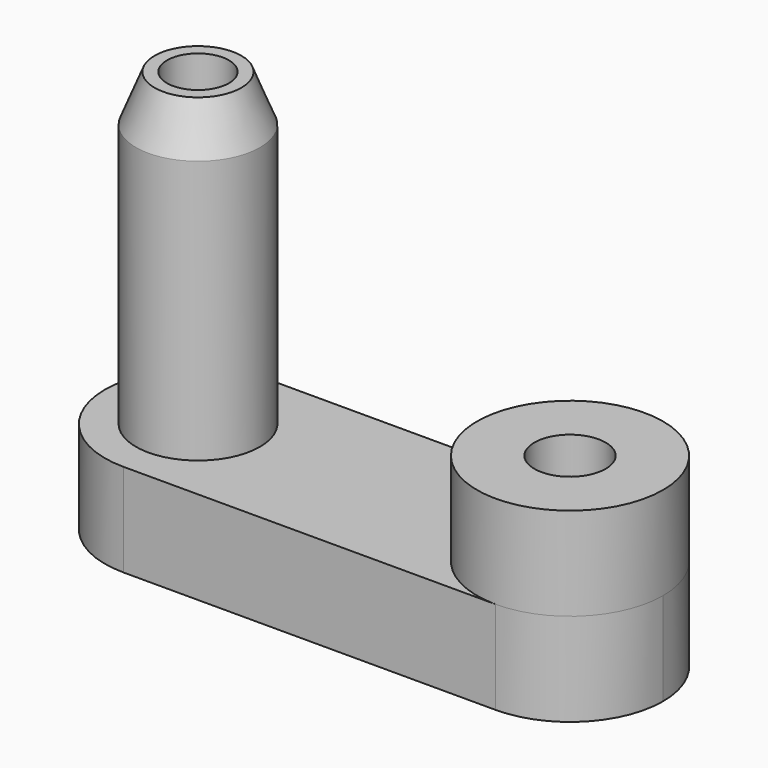
from build123d import *

# Parameters (mm, degrees)
F0_W      = 18
F0_H      = 6
F1_DEPTH  = 3
F2_R      = 3
F2_R_2    = 2
F3_DEPTH  = 10
F4_R      = 1
F4_R_2    = 1.15
F5_DEPTH  = 20
F6_SIZE2  = 1.5
F6_SIZE   = 0.6
F7_W      = 11.6012076614
F7_H      = 11.8295210414
F8_DEPTH  = 7
F9_R      = 2.9999
F10_R     = 2.55
F10_R_2   = 1
F11_DEPTH = 1.5


# Not quite as in the source:
# - a fillet or chamfer is up to 0.001 mm smaller than in the source, because OpenCascade refuses the exact size


with BuildPart() as f1:
    # F0 (on Top) → F1 (new body)
    with BuildSketch(Plane.XY):
        with Locations((1.8924829921, 0)):
            Rectangle(F0_W, F0_H)
    extrude(amount=F1_DEPTH)

    # F2 (on face) → F3 (join)
    with BuildSketch(Plane.XY.offset(3)):
        with Locations((7.8924829921, 0)):
            Circle(F2_R)
        with Locations((-4.1075170079, 0)):
            Circle(F2_R_2)
    extrude(amount=F3_DEPTH)

    # F4 (on face) → F5 (cut)
    with BuildSketch(Plane.XY.offset(13)):
        with Locations((-4.1075170079, 0)):
            Circle(F4_R)
        with Locations((7.8924829921, 0)):
            Circle(F4_R_2)
    extrude(amount=-F5_DEPTH, mode=Mode.SUBTRACT)

    # F6
    f6_edges = [f1.edges().sort_by_distance(p)[0] for p in [
        (-6.107517, 0, 13),
    ]]
    f6_side = f1.faces().sort_by_distance((-6.050948, 0, 13))[0]
    chamfer(f6_edges, length=F6_SIZE, length2=F6_SIZE2, reference=f6_side)

    # F7 (on face) → F8 (cut)
    with BuildSketch(Plane.XY.offset(13)):
        with Locations((7.5882198871, -0.5373002496)):
            Rectangle(F7_W, F7_H)
    extrude(amount=-F8_DEPTH, mode=Mode.SUBTRACT)

    # F9 (radius 3 in the source; OpenCascade refuses exactly that, so slightly less here)
    f9_edges = [f1.edges().sort_by_distance(p)[0] for p in [
        (10.892483, -3, 1.5),
        (10.892483, 3, 1.5),
        (-7.107517, 3, 1.5),
        (-7.107517, -3, 1.5),
    ]]
    fillet(f9_edges, radius=F9_R)

    # F10 (on face) → F11 (cut)
    with BuildSketch(Plane(origin=(0, 0, 0), x_dir=(1, 0, 0), z_dir=(0, 0, -1))):
        with Locations((-4.1075170079, 0)):
            Circle(F10_R)
        with Locations((-4.1075170079, 0)):
            Circle(F10_R_2, mode=Mode.SUBTRACT)
    extrude(amount=-F11_DEPTH, mode=Mode.SUBTRACT)


solid = f1.part
